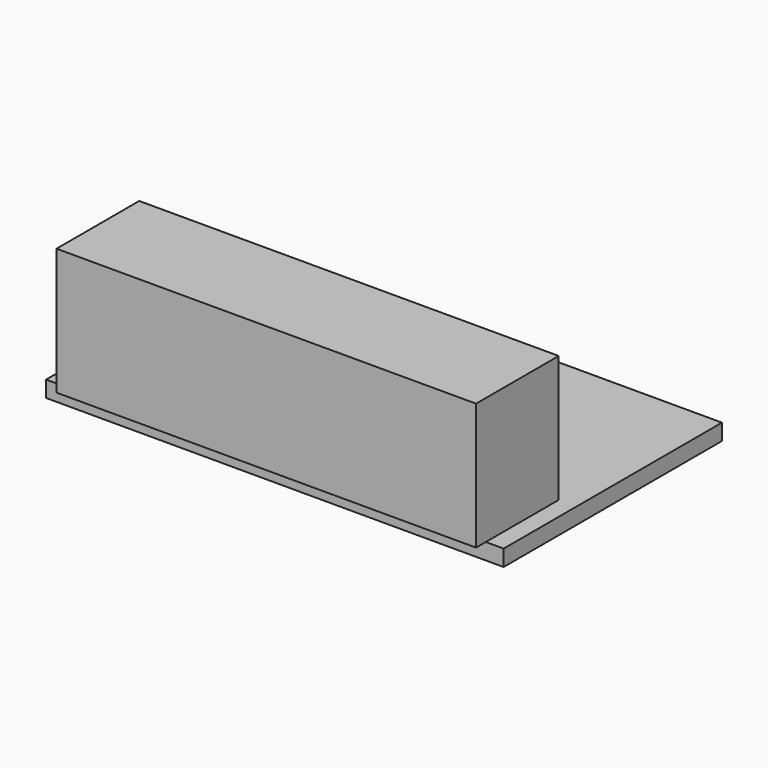
from build123d import *

# Parameters (mm, degrees)
F0_W     = 56.3871189952
F0_H     = 33.6253512651
F1_DEPTH = 2
F2_W     = 51.7
F2_H     = 11.2356165416
F3_DEPTH = 15.62
F4_W     = 51.7
F4_H     = 15.62
F5_DEPTH = 1.5


# Not quite as in the source:
# - a feature of the source that left no trace in its solid (it failed there, or was rolled back) is left out


with BuildPart() as f1:
    # F0 (on Top) → F1 (new body)
    with BuildSketch(Plane.XY):
        with Locations((-6.0005225241, 2.1580690518)):
            Rectangle(F0_W, F0_H)
    extrude(amount=F1_DEPTH)

    # F2 (on face) → F3 (join)
    with BuildSketch(Plane.XY.offset(2)):
        with Locations((-5.8556830972, -9.0367983099)):
            Rectangle(F2_W, F2_H)
    extrude(amount=F3_DEPTH)

    # F4 (on face) → F5 (join)
    with BuildSketch(Plane.XZ.offset(14.6546065807)):
        with Locations((-5.8556830972, 9.81)):
            Rectangle(F4_W, F4_H)
    extrude(amount=F5_DEPTH)


solid = f1.part
